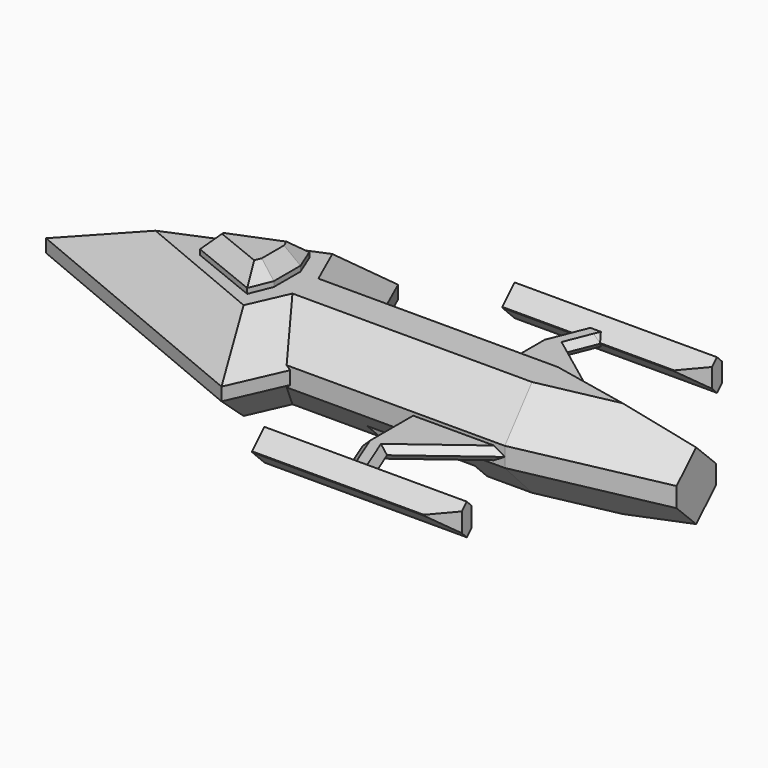
from build123d import *

# Parameters (mm, degrees)
F1_DEPTH      = 37.5
F2_SIZE       = 32.5
F3_DEPTH      = 5
F4_DEPTH      = 12.5
F5_SIZE       = 30
F6_SIZE       = 4.99999
F7_T1_DEPTH   = 216.7867093217
F7_T6_DEPTH   = 216.7867093217
F7_T12_DEPTH  = 216.7867093217
F7_T19_DEPTH  = 216.7867093217
F7_T25_DEPTH  = 216.7867093217
F7_T32_DEPTH  = 216.7867093217
F7_T38_DEPTH  = 216.7867093217
F7_T45_DEPTH  = 216.7867093217
F7_T51_DEPTH  = 216.7867093217
F7_T58_DEPTH  = 216.7867093217
F7_T64_DEPTH  = 216.7867093217
F7_T71_DEPTH  = 216.7867093217
F7_T77_DEPTH  = 216.7867093217
F7_T84_DEPTH  = 216.7867093217
F7_T90_DEPTH  = 216.7867093217
F7_T97_DEPTH  = 216.7867093217
F7_T103_DEPTH = 216.7867093217
F7_T110_DEPTH = 216.7867093217
F7_T116_DEPTH = 216.7867093217
F7_T123_DEPTH = 216.7867093217
F7_T129_DEPTH = 216.7867093217
F7_T136_DEPTH = 216.7867093217
F7_T142_DEPTH = 216.7867093217
F7_T149_DEPTH = 216.7867093217
F7_T155_DEPTH = 216.7867093217
F10_DEPTH     = 15
F11_SIZE      = 11
F13_W         = 82.6045945287
F13_H         = 48.8392151892
F14_DEPTH     = 25


# Not quite as in the source:
# - a fillet or chamfer that OpenCascade refuses, or shapes differently, is made with other operations: its cross-section is extruded or revolved along the edge and cut away or added
# - a fillet or chamfer is up to 0.001 mm smaller than in the source, because OpenCascade refuses the exact size
# - a feature names something its author has since deleted; it is built from what else it names


with BuildPart() as f1:
    # F0 (on Top) → F1 (new body, symmetric)
    with BuildSketch(Plane.XY):
        Polygon((-106.6587882222, 84.9056603774), (-309.4889769014, 0), (-106.6587882222, -84.9056603774), (-87.7908636939, -42.4528301887), (1.8317778155, -42.4528301887), (77.3034759288, -42.4528301887), (190.5110230986, -18.8679245283), (190.5110230986, 18.8679245283), (77.3034759288, 42.4528301887), (1.8317778155, 42.4528301887), (-87.7908636939, 42.4528301887), align=None)
    extrude(amount=F1_DEPTH, both=True)

    # F2
    f2_edges = [f1.edges().sort_by_distance(p)[0] for p in [
        (-208.073883, 42.45283, -37.5),
        (-208.073883, 42.45283, 37.5),
        (-208.073883, -42.45283, 37.5),
        (-208.073883, -42.45283, -37.5),
        (-97.224826, -63.679245, 37.5),
        (-97.224826, -63.679245, -37.5),
        (-97.224826, 63.679245, 37.5),
        (-97.224826, 63.679245, -37.5),
    ]]
    chamfer(f2_edges, length=F2_SIZE)

    # F0 (on Top) → F3 (join, symmetric)
    with BuildSketch(Plane.XY):
        Polygon((77.3034759288, -42.4528301887), (1.8317778155, -42.4528301887), (1.8317778155, -84.9056603774), (11.2657400797, -108.4905660377), (30.133664608, -108.4905660377), (20.6997023439, -84.9056603774), align=None)
        Polygon((1.8317778155, 84.9056603774), (1.8317778155, 42.4528301887), (77.3034759288, 42.4528301887), (20.6997023439, 84.9056603774), (30.133664608, 108.4905660377), (11.2657400797, 108.4905660377), align=None)
    extrude(amount=F3_DEPTH, both=True)

    # F0 (on Top) → F4 (join, symmetric)
    with BuildSketch(Plane.XY):
        Polygon((-45.3380335052, 108.4905660377), (11.2657400797, 108.4905660377), (30.133664608, 108.4905660377), (86.7374381929, 108.4905660377), (110.3223438533, 115.5660377358), (110.3223438533, 125), (86.7374381929, 132.0754716981), (-45.3380335052, 132.0754716981), align=None)
        Polygon((30.133664608, -108.4905660377), (11.2657400797, -108.4905660377), (-45.3380335052, -108.4905660377), (-45.3380335052, -132.0754716981), (86.7374381929, -132.0754716981), (110.3223438533, -125), (110.3223438533, -115.5660377358), (86.7374381929, -108.4905660377), align=None)
    extrude(amount=F4_DEPTH, both=True)

    # F5 (call 1 of 4: OpenCascade refuses the feature's edges together)
    f5_edges = [f1.edges().sort_by_distance(p)[0] for p in [
        (133.90725, 30.660377, -37.5),
        (-23.026354, 42.45283, -37.5),
    ]]
    chamfer(f5_edges, length=F5_SIZE)

    # F5#2 (call 2 of 4)
    f5_2_edges = [f1.edges().sort_by_distance(p)[0] for p in [
        (133.90725, 30.660377, 37.5),
        (-23.026354, 42.45283, 37.5),
    ]]
    chamfer(f5_2_edges, length=F5_SIZE)

    # F5#3 (call 3 of 4)
    f5_3_edges = [f1.edges().sort_by_distance(p)[0] for p in [
        (133.90725, -30.660377, 37.5),
        (-23.026354, -42.45283, 37.5),
    ]]
    chamfer(f5_3_edges, length=F5_SIZE)

    # F5#4 (call 4 of 4)
    f5_4_edges = [f1.edges().sort_by_distance(p)[0] for p in [
        (133.90725, -30.660377, -37.5),
        (-23.026354, -42.45283, -37.5),
    ]]
    chamfer(f5_4_edges, length=F5_SIZE)

    # F6 (size 5 in the source; OpenCascade refuses exactly that, so slightly less here)
    f6_edges = [f1.edges().sort_by_distance(p)[0] for p in [
        (1.831778, 63.679245, 5),
        (1.831778, 63.679245, -5),
        (49.001589, 63.679245, -5),
        (6.548759, 96.698113, 5),
        (6.548759, 96.698113, -5),
        (25.416683, 96.698113, -5),
        (25.416683, 96.698113, 5),
        (49.001589, -63.679245, -5),
        (1.831778, -63.679245, -5),
        (6.548759, -96.698113, -5),
        (25.416683, -96.698113, -5),
        (1.831778, -63.679245, 5),
        (6.548759, -96.698113, 5),
        (49.001589, -63.679245, 5),
        (25.416683, -96.698113, 5),
    ]]
    chamfer(f6_edges, length=F6_SIZE)

    # F7: chamfer of 12.2 on 8 edges, made by hand

    # F7_s2 → F7_t1 (cut)
    with BuildSketch(Plane.YZ.offset(-76.7125659584)):
        Polygon((-119.8754716981, 12.5), (-132.0754716981, 0.3), (-132.0754716981, 12.5), align=None)
        Polygon((-119.8754716981, -12.5), (-132.0754716981, -0.3), (-132.0754716981, -12.5), align=None)
        Polygon((119.8754716981, -12.5), (132.0754716981, -0.3), (132.0754716981, -12.5), align=None)
        Polygon((119.8754716981, 12.5), (132.0754716981, 0.3), (132.0754716981, 12.5), align=None)
    extrude(amount=F7_T1_DEPTH, mode=Mode.SUBTRACT)


with BuildPart() as f7_tool4:
    # F7_s5 → F7_t6 (new body)
    with BuildSketch(Plane.YZ.offset(140.0741433633)):
        Polygon((-108.4905660377, 0.3), (-120.6905660377, 12.5), (-108.4905660377, 12.5), align=None)
    extrude(amount=-F7_T6_DEPTH)

    split(bisect_by=Plane.XY.offset(5), keep=Keep.BOTTOM)

    split(bisect_by=Plane(origin=(-5.7166168262, -2.2866467305, -6.1569847497), x_dir=(-0.3713906764, 0.9284766909, 0), z_dir=(0.6565321643, 0.2626128657, 0.7071067812)), keep=Keep.TOP)


with BuildPart() as f1_1:
    add(f1.part)

    # F7_t3: cut F7_tool4
    add(f7_tool4.part, mode=Mode.SUBTRACT)


with BuildPart() as f7_tool10:
    # F7_s11 → F7_t12 (new body)
    with BuildSketch(Plane.YZ.offset(140.0741433633)):
        Polygon((-108.4905660377, 0.3), (-120.6905660377, 12.5), (-108.4905660377, 12.5), align=None)
    extrude(amount=-F7_T12_DEPTH)

    split(bisect_by=Plane.XY.offset(5), keep=Keep.TOP)

    split(bisect_by=Plane(origin=(-5.7166168262, -2.2866467305, -6.1569847497), x_dir=(-0.3713906764, 0.9284766909, 0), z_dir=(0.6565321643, 0.2626128657, 0.7071067812)), keep=Keep.TOP)

    split(bisect_by=Plane(origin=(-13.8493522007, -5.5397408803, 14.9162088146), x_dir=(-0.3713906764, 0.9284766909, 0), z_dir=(0.6565321643, 0.2626128657, -0.7071067812)), keep=Keep.TOP)


with BuildPart() as f1_2:
    add(f1_1.part)

    # F7_t9: cut F7_tool10
    add(f7_tool10.part, mode=Mode.SUBTRACT)


with BuildPart() as f7_tool17:
    # F7_s18 → F7_t19 (new body)
    with BuildSketch(Plane.YZ.offset(140.0741433633)):
        Polygon((-108.4905660377, 0.3), (-120.6905660377, 12.5), (-108.4905660377, 12.5), align=None)
    extrude(amount=-F7_T19_DEPTH)

    split(bisect_by=Plane(origin=(-5.7166168262, -2.2866467305, -6.1569847497), x_dir=(-0.3713906764, 0.9284766909, 0), z_dir=(0.6565321643, 0.2626128657, 0.7071067812)), keep=Keep.TOP)

    split(bisect_by=Plane(origin=(-13.8493522007, -5.5397408803, 14.9162088146), x_dir=(0.3713906764, -0.9284766909, 0), z_dir=(-0.6565321643, -0.2626128657, 0.7071067812)), keep=Keep.TOP)


with BuildPart() as f1_3:
    add(f1_2.part)

    # F7_t16: cut F7_tool17
    add(f7_tool17.part, mode=Mode.SUBTRACT)


with BuildPart() as f7_tool23:
    # F7_s24 → F7_t25 (new body)
    with BuildSketch(Plane.YZ.offset(140.0741433633)):
        Polygon((-108.4905660377, 0.3), (-120.6905660377, 12.5), (-108.4905660377, 12.5), align=None)
    extrude(amount=-F7_T25_DEPTH)

    split(bisect_by=Plane.XY.offset(5), keep=Keep.TOP)

    split(bisect_by=Plane(origin=(-5.7166168262, -2.2866467305, -6.1569847497), x_dir=(0.3713906764, -0.9284766909, 0), z_dir=(-0.6565321643, -0.2626128657, -0.7071067812)), keep=Keep.TOP)

    split(bisect_by=Plane(origin=(-13.8493522007, -5.5397408803, 14.9162088146), x_dir=(-0.3713906764, 0.9284766909, 0), z_dir=(0.6565321643, 0.2626128657, -0.7071067812)), keep=Keep.TOP)


with BuildPart() as f1_4:
    add(f1_3.part)

    # F7_t22: cut F7_tool23
    add(f7_tool23.part, mode=Mode.SUBTRACT)


with BuildPart() as f7_tool30:
    # F7_s31 → F7_t32 (new body)
    with BuildSketch(Plane.YZ.offset(140.0741433633)):
        Polygon((-108.4905660377, 0.3), (-120.6905660377, 12.5), (-108.4905660377, 12.5), align=None)
    extrude(amount=-F7_T32_DEPTH)

    split(bisect_by=Plane.XY.offset(5), keep=Keep.BOTTOM)

    split(bisect_by=Plane(origin=(-13.8493522007, -5.5397408803, 14.9162088146), x_dir=(0.3713906764, -0.9284766909, 0), z_dir=(-0.6565321643, -0.2626128657, 0.7071067812)), keep=Keep.TOP)


with BuildPart() as f1_5:
    add(f1_4.part)

    # F7_t29: cut F7_tool30
    add(f7_tool30.part, mode=Mode.SUBTRACT)


with BuildPart() as f7_tool36:
    # F7_s37 → F7_t38 (new body)
    with BuildSketch(Plane.YZ.offset(140.0741433633)):
        Polygon((-108.4905660377, 0.3), (-120.6905660377, 12.5), (-108.4905660377, 12.5), align=None)
    extrude(amount=-F7_T38_DEPTH)

    split(bisect_by=Plane.XY.offset(5), keep=Keep.TOP)

    split(bisect_by=Plane(origin=(-5.7166168262, -2.2866467305, -6.1569847497), x_dir=(0.3713906764, -0.9284766909, 0), z_dir=(-0.6565321643, -0.2626128657, -0.7071067812)), keep=Keep.TOP)

    split(bisect_by=Plane(origin=(-13.8493522007, -5.5397408803, 14.9162088146), x_dir=(0.3713906764, -0.9284766909, 0), z_dir=(-0.6565321643, -0.2626128657, 0.7071067812)), keep=Keep.TOP)


with BuildPart() as f1_6:
    add(f1_5.part)

    # F7_t35: cut F7_tool36
    add(f7_tool36.part, mode=Mode.SUBTRACT)


with BuildPart() as f7_tool43:
    # F7_s44 → F7_t45 (new body)
    with BuildSketch(Plane.YZ.offset(140.0741433633)):
        Polygon((-108.4905660377, -0.3), (-120.6905660377, -12.5), (-108.4905660377, -12.5), align=None)
    extrude(amount=-F7_T45_DEPTH)

    split(bisect_by=Plane.XY.offset(-5), keep=Keep.TOP)

    split(bisect_by=Plane(origin=(-5.7166168262, -2.2866467305, 6.1569847497), x_dir=(-0.3713906764, 0.9284766909, 0), z_dir=(0.6565321643, 0.2626128657, -0.7071067812)), keep=Keep.TOP)


with BuildPart() as f1_7:
    add(f1_6.part)

    # F7_t42: cut F7_tool43
    add(f7_tool43.part, mode=Mode.SUBTRACT)


with BuildPart() as f7_tool49:
    # F7_s50 → F7_t51 (new body)
    with BuildSketch(Plane.YZ.offset(140.0741433633)):
        Polygon((-108.4905660377, -0.3), (-120.6905660377, -12.5), (-108.4905660377, -12.5), align=None)
    extrude(amount=-F7_T51_DEPTH)

    split(bisect_by=Plane.XY.offset(-5), keep=Keep.BOTTOM)

    split(bisect_by=Plane(origin=(-5.7166168262, -2.2866467305, 6.1569847497), x_dir=(-0.3713906764, 0.9284766909, 0), z_dir=(0.6565321643, 0.2626128657, -0.7071067812)), keep=Keep.TOP)

    split(bisect_by=Plane(origin=(-13.8493522007, -5.5397408803, -14.9162088146), x_dir=(-0.3713906764, 0.9284766909, 0), z_dir=(0.6565321643, 0.2626128657, 0.7071067812)), keep=Keep.TOP)


with BuildPart() as f1_8:
    add(f1_7.part)

    # F7_t48: cut F7_tool49
    add(f7_tool49.part, mode=Mode.SUBTRACT)


with BuildPart() as f7_tool56:
    # F7_s57 → F7_t58 (new body)
    with BuildSketch(Plane.YZ.offset(140.0741433633)):
        Polygon((-108.4905660377, -0.3), (-120.6905660377, -12.5), (-108.4905660377, -12.5), align=None)
    extrude(amount=-F7_T58_DEPTH)

    split(bisect_by=Plane(origin=(-5.7166168262, -2.2866467305, 6.1569847497), x_dir=(-0.3713906764, 0.9284766909, 0), z_dir=(0.6565321643, 0.2626128657, -0.7071067812)), keep=Keep.TOP)

    split(bisect_by=Plane(origin=(-13.8493522007, -5.5397408803, -14.9162088146), x_dir=(0.3713906764, -0.9284766909, 0), z_dir=(-0.6565321643, -0.2626128657, -0.7071067812)), keep=Keep.TOP)


with BuildPart() as f1_9:
    add(f1_8.part)

    # F7_t55: cut F7_tool56
    add(f7_tool56.part, mode=Mode.SUBTRACT)


with BuildPart() as f7_tool62:
    # F7_s63 → F7_t64 (new body)
    with BuildSketch(Plane.YZ.offset(140.0741433633)):
        Polygon((-108.4905660377, -0.3), (-120.6905660377, -12.5), (-108.4905660377, -12.5), align=None)
    extrude(amount=-F7_T64_DEPTH)

    split(bisect_by=Plane.XY.offset(-5), keep=Keep.BOTTOM)

    split(bisect_by=Plane(origin=(-5.7166168262, -2.2866467305, 6.1569847497), x_dir=(0.3713906764, -0.9284766909, 0), z_dir=(-0.6565321643, -0.2626128657, 0.7071067812)), keep=Keep.TOP)

    split(bisect_by=Plane(origin=(-13.8493522007, -5.5397408803, -14.9162088146), x_dir=(-0.3713906764, 0.9284766909, 0), z_dir=(0.6565321643, 0.2626128657, 0.7071067812)), keep=Keep.TOP)


with BuildPart() as f1_10:
    add(f1_9.part)

    # F7_t61: cut F7_tool62
    add(f7_tool62.part, mode=Mode.SUBTRACT)


with BuildPart() as f7_tool69:
    # F7_s70 → F7_t71 (new body)
    with BuildSketch(Plane.YZ.offset(140.0741433633)):
        Polygon((-108.4905660377, -0.3), (-120.6905660377, -12.5), (-108.4905660377, -12.5), align=None)
    extrude(amount=-F7_T71_DEPTH)

    split(bisect_by=Plane.XY.offset(-5), keep=Keep.TOP)

    split(bisect_by=Plane(origin=(-13.8493522007, -5.5397408803, -14.9162088146), x_dir=(0.3713906764, -0.9284766909, 0), z_dir=(-0.6565321643, -0.2626128657, -0.7071067812)), keep=Keep.TOP)


with BuildPart() as f1_11:
    add(f1_10.part)

    # F7_t68: cut F7_tool69
    add(f7_tool69.part, mode=Mode.SUBTRACT)


with BuildPart() as f7_tool75:
    # F7_s76 → F7_t77 (new body)
    with BuildSketch(Plane.YZ.offset(140.0741433633)):
        Polygon((-108.4905660377, -0.3), (-120.6905660377, -12.5), (-108.4905660377, -12.5), align=None)
    extrude(amount=-F7_T77_DEPTH)

    split(bisect_by=Plane.XY.offset(-5), keep=Keep.BOTTOM)

    split(bisect_by=Plane(origin=(-5.7166168262, -2.2866467305, 6.1569847497), x_dir=(0.3713906764, -0.9284766909, 0), z_dir=(-0.6565321643, -0.2626128657, 0.7071067812)), keep=Keep.TOP)

    split(bisect_by=Plane(origin=(-13.8493522007, -5.5397408803, -14.9162088146), x_dir=(0.3713906764, -0.9284766909, 0), z_dir=(-0.6565321643, -0.2626128657, -0.7071067812)), keep=Keep.TOP)


with BuildPart() as f1_12:
    add(f1_11.part)

    # F7_t74: cut F7_tool75
    add(f7_tool75.part, mode=Mode.SUBTRACT)


with BuildPart() as f7_tool82:
    # F7_s83 → F7_t84 (new body)
    with BuildSketch(Plane.YZ.offset(-76.7125659584)):
        Polygon((108.4905660377, 0.3), (120.6905660377, 12.5), (108.4905660377, 12.5), align=None)
    extrude(amount=F7_T84_DEPTH)

    split(bisect_by=Plane.XY.offset(5), keep=Keep.BOTTOM)

    split(bisect_by=Plane(origin=(-13.8493522007, 5.5397408803, 14.9162088146), x_dir=(-0.3713906764, -0.9284766909, 0), z_dir=(-0.6565321643, 0.2626128657, 0.7071067812)), keep=Keep.TOP)


with BuildPart() as f1_13:
    add(f1_12.part)

    # F7_t81: cut F7_tool82
    add(f7_tool82.part, mode=Mode.SUBTRACT)


with BuildPart() as f7_tool88:
    # F7_s89 → F7_t90 (new body)
    with BuildSketch(Plane.YZ.offset(-76.7125659584)):
        Polygon((108.4905660377, 0.3), (120.6905660377, 12.5), (108.4905660377, 12.5), align=None)
    extrude(amount=F7_T90_DEPTH)

    split(bisect_by=Plane.XY.offset(5), keep=Keep.TOP)

    split(bisect_by=Plane(origin=(-5.7166168262, 2.2866467305, -6.1569847497), x_dir=(-0.3713906764, -0.9284766909, 0), z_dir=(-0.6565321643, 0.2626128657, -0.7071067812)), keep=Keep.TOP)

    split(bisect_by=Plane(origin=(-13.8493522007, 5.5397408803, 14.9162088146), x_dir=(-0.3713906764, -0.9284766909, 0), z_dir=(-0.6565321643, 0.2626128657, 0.7071067812)), keep=Keep.TOP)


with BuildPart() as f1_14:
    add(f1_13.part)

    # F7_t87: cut F7_tool88
    add(f7_tool88.part, mode=Mode.SUBTRACT)


with BuildPart() as f7_tool95:
    # F7_s96 → F7_t97 (new body)
    with BuildSketch(Plane.YZ.offset(-76.7125659584)):
        Polygon((108.4905660377, 0.3), (120.6905660377, 12.5), (108.4905660377, 12.5), align=None)
    extrude(amount=F7_T97_DEPTH)

    split(bisect_by=Plane(origin=(-5.7166168262, 2.2866467305, -6.1569847497), x_dir=(0.3713906764, 0.9284766909, 0), z_dir=(0.6565321643, -0.2626128657, 0.7071067812)), keep=Keep.TOP)

    split(bisect_by=Plane(origin=(-13.8493522007, 5.5397408803, 14.9162088146), x_dir=(-0.3713906764, -0.9284766909, 0), z_dir=(-0.6565321643, 0.2626128657, 0.7071067812)), keep=Keep.TOP)


with BuildPart() as f1_15:
    add(f1_14.part)

    # F7_t94: cut F7_tool95
    add(f7_tool95.part, mode=Mode.SUBTRACT)


with BuildPart() as f7_tool101:
    # F7_s102 → F7_t103 (new body)
    with BuildSketch(Plane.YZ.offset(-76.7125659584)):
        Polygon((108.4905660377, 0.3), (120.6905660377, 12.5), (108.4905660377, 12.5), align=None)
    extrude(amount=F7_T103_DEPTH)

    split(bisect_by=Plane.XY.offset(5), keep=Keep.TOP)

    split(bisect_by=Plane(origin=(-5.7166168262, 2.2866467305, -6.1569847497), x_dir=(-0.3713906764, -0.9284766909, 0), z_dir=(-0.6565321643, 0.2626128657, -0.7071067812)), keep=Keep.TOP)

    split(bisect_by=Plane(origin=(-13.8493522007, 5.5397408803, 14.9162088146), x_dir=(0.3713906764, 0.9284766909, 0), z_dir=(0.6565321643, -0.2626128657, -0.7071067812)), keep=Keep.TOP)


with BuildPart() as f1_16:
    add(f1_15.part)

    # F7_t100: cut F7_tool101
    add(f7_tool101.part, mode=Mode.SUBTRACT)


with BuildPart() as f7_tool108:
    # F7_s109 → F7_t110 (new body)
    with BuildSketch(Plane.YZ.offset(-76.7125659584)):
        Polygon((108.4905660377, 0.3), (120.6905660377, 12.5), (108.4905660377, 12.5), align=None)
    extrude(amount=F7_T110_DEPTH)

    split(bisect_by=Plane.XY.offset(5), keep=Keep.BOTTOM)

    split(bisect_by=Plane(origin=(-5.7166168262, 2.2866467305, -6.1569847497), x_dir=(0.3713906764, 0.9284766909, 0), z_dir=(0.6565321643, -0.2626128657, 0.7071067812)), keep=Keep.TOP)


with BuildPart() as f1_17:
    add(f1_16.part)

    # F7_t107: cut F7_tool108
    add(f7_tool108.part, mode=Mode.SUBTRACT)


with BuildPart() as f7_tool114:
    # F7_s115 → F7_t116 (new body)
    with BuildSketch(Plane.YZ.offset(-76.7125659584)):
        Polygon((108.4905660377, 0.3), (120.6905660377, 12.5), (108.4905660377, 12.5), align=None)
    extrude(amount=F7_T116_DEPTH)

    split(bisect_by=Plane.XY.offset(5), keep=Keep.TOP)

    split(bisect_by=Plane(origin=(-5.7166168262, 2.2866467305, -6.1569847497), x_dir=(0.3713906764, 0.9284766909, 0), z_dir=(0.6565321643, -0.2626128657, 0.7071067812)), keep=Keep.TOP)

    split(bisect_by=Plane(origin=(-13.8493522007, 5.5397408803, 14.9162088146), x_dir=(0.3713906764, 0.9284766909, 0), z_dir=(0.6565321643, -0.2626128657, -0.7071067812)), keep=Keep.TOP)


with BuildPart() as f1_18:
    add(f1_17.part)

    # F7_t113: cut F7_tool114
    add(f7_tool114.part, mode=Mode.SUBTRACT)


with BuildPart() as f7_tool121:
    # F7_s122 → F7_t123 (new body)
    with BuildSketch(Plane.YZ.offset(-76.7125659584)):
        Polygon((108.4905660377, -0.3), (120.6905660377, -12.5), (108.4905660377, -12.5), align=None)
    extrude(amount=F7_T123_DEPTH)

    split(bisect_by=Plane.XY.offset(-5), keep=Keep.TOP)

    split(bisect_by=Plane(origin=(-13.8493522007, 5.5397408803, -14.9162088146), x_dir=(-0.3713906764, -0.9284766909, 0), z_dir=(-0.6565321643, 0.2626128657, -0.7071067812)), keep=Keep.TOP)


with BuildPart() as f1_19:
    add(f1_18.part)

    # F7_t120: cut F7_tool121
    add(f7_tool121.part, mode=Mode.SUBTRACT)


with BuildPart() as f7_tool127:
    # F7_s128 → F7_t129 (new body)
    with BuildSketch(Plane.YZ.offset(-76.7125659584)):
        Polygon((108.4905660377, -0.3), (120.6905660377, -12.5), (108.4905660377, -12.5), align=None)
    extrude(amount=F7_T129_DEPTH)

    split(bisect_by=Plane.XY.offset(-5), keep=Keep.BOTTOM)

    split(bisect_by=Plane(origin=(-5.7166168262, 2.2866467305, 6.1569847497), x_dir=(-0.3713906764, -0.9284766909, 0), z_dir=(-0.6565321643, 0.2626128657, 0.7071067812)), keep=Keep.TOP)

    split(bisect_by=Plane(origin=(-13.8493522007, 5.5397408803, -14.9162088146), x_dir=(-0.3713906764, -0.9284766909, 0), z_dir=(-0.6565321643, 0.2626128657, -0.7071067812)), keep=Keep.TOP)


with BuildPart() as f1_20:
    add(f1_19.part)

    # F7_t126: cut F7_tool127
    add(f7_tool127.part, mode=Mode.SUBTRACT)


with BuildPart() as f7_tool134:
    # F7_s135 → F7_t136 (new body)
    with BuildSketch(Plane.YZ.offset(-76.7125659584)):
        Polygon((108.4905660377, -0.3), (120.6905660377, -12.5), (108.4905660377, -12.5), align=None)
    extrude(amount=F7_T136_DEPTH)

    split(bisect_by=Plane(origin=(-5.7166168262, 2.2866467305, 6.1569847497), x_dir=(0.3713906764, 0.9284766909, 0), z_dir=(0.6565321643, -0.2626128657, -0.7071067812)), keep=Keep.TOP)

    split(bisect_by=Plane(origin=(-13.8493522007, 5.5397408803, -14.9162088146), x_dir=(-0.3713906764, -0.9284766909, 0), z_dir=(-0.6565321643, 0.2626128657, -0.7071067812)), keep=Keep.TOP)


with BuildPart() as f1_21:
    add(f1_20.part)

    # F7_t133: cut F7_tool134
    add(f7_tool134.part, mode=Mode.SUBTRACT)


with BuildPart() as f7_tool140:
    # F7_s141 → F7_t142 (new body)
    with BuildSketch(Plane.YZ.offset(-76.7125659584)):
        Polygon((108.4905660377, -0.3), (120.6905660377, -12.5), (108.4905660377, -12.5), align=None)
    extrude(amount=F7_T142_DEPTH)

    split(bisect_by=Plane.XY.offset(-5), keep=Keep.BOTTOM)

    split(bisect_by=Plane(origin=(-5.7166168262, 2.2866467305, 6.1569847497), x_dir=(-0.3713906764, -0.9284766909, 0), z_dir=(-0.6565321643, 0.2626128657, 0.7071067812)), keep=Keep.TOP)

    split(bisect_by=Plane(origin=(-13.8493522007, 5.5397408803, -14.9162088146), x_dir=(0.3713906764, 0.9284766909, 0), z_dir=(0.6565321643, -0.2626128657, 0.7071067812)), keep=Keep.TOP)


with BuildPart() as f1_22:
    add(f1_21.part)

    # F7_t139: cut F7_tool140
    add(f7_tool140.part, mode=Mode.SUBTRACT)


with BuildPart() as f7_tool147:
    # F7_s148 → F7_t149 (new body)
    with BuildSketch(Plane.YZ.offset(-76.7125659584)):
        Polygon((108.4905660377, -0.3), (120.6905660377, -12.5), (108.4905660377, -12.5), align=None)
    extrude(amount=F7_T149_DEPTH)

    split(bisect_by=Plane.XY.offset(-5), keep=Keep.TOP)

    split(bisect_by=Plane(origin=(-5.7166168262, 2.2866467305, 6.1569847497), x_dir=(0.3713906764, 0.9284766909, 0), z_dir=(0.6565321643, -0.2626128657, -0.7071067812)), keep=Keep.TOP)


with BuildPart() as f1_23:
    add(f1_22.part)

    # F7_t146: cut F7_tool147
    add(f7_tool147.part, mode=Mode.SUBTRACT)


with BuildPart() as f7_tool153:
    # F7_s154 → F7_t155 (new body)
    with BuildSketch(Plane.YZ.offset(-76.7125659584)):
        Polygon((108.4905660377, -0.3), (120.6905660377, -12.5), (108.4905660377, -12.5), align=None)
    extrude(amount=F7_T155_DEPTH)

    split(bisect_by=Plane.XY.offset(-5), keep=Keep.BOTTOM)

    split(bisect_by=Plane(origin=(-5.7166168262, 2.2866467305, 6.1569847497), x_dir=(0.3713906764, 0.9284766909, 0), z_dir=(0.6565321643, -0.2626128657, -0.7071067812)), keep=Keep.TOP)

    split(bisect_by=Plane(origin=(-13.8493522007, 5.5397408803, -14.9162088146), x_dir=(0.3713906764, 0.9284766909, 0), z_dir=(0.6565321643, -0.2626128657, 0.7071067812)), keep=Keep.TOP)


with BuildPart() as f1_24:
    add(f1_23.part)

    # F7_t152: cut F7_tool153
    add(f7_tool153.part, mode=Mode.SUBTRACT)

    # F9 (on offset) → F10 (join)
    with BuildSketch(Plane.XY.offset(37.5)):
        Polygon((-184.6017837524, 8.1398682669), (-184.6017837524, -8.1398682669), (-130.9389472008, -29.8461858183), (-124.052836571, -12.8221913831), (-124.052836571, 12.8221913831), (-130.9389472008, 29.8461858183), align=None)
    extrude(amount=F10_DEPTH)

    # F11
    f11_edges = [f1_24.edges().sort_by_distance(p)[0] for p in [
        (-157.770365, 18.993027, 52.5),
        (-184.601784, 0, 52.5),
        (-157.770365, -18.993027, 52.5),
        (-127.495892, -21.334189, 52.5),
        (-124.052837, 0, 52.5),
        (-127.495892, 21.334189, 52.5),
    ]]
    chamfer(f11_edges, length=F11_SIZE)

    # F13 (on offset) → F14 (cut)
    with BuildSketch(Plane.XY.offset(-12.5)):
        with Locations((-1.6054697335, 0)):
            Rectangle(F13_W, F13_H)
    extrude(amount=-F14_DEPTH, mode=Mode.SUBTRACT)


solid = f1_24.part
